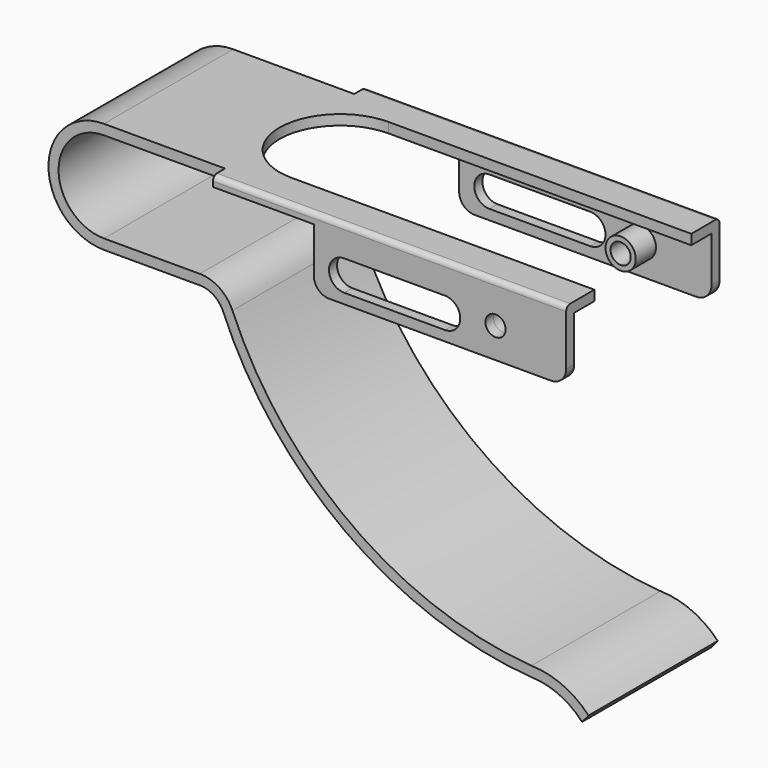
from build123d import *

# Parameters (mm, degrees)
F1_DEPTH  = 16
F2_W      = 70
F2_H      = 3
F3_DEPTH  = 2
F4_W      = 50
F4_H      = 14
F5_DEPTH  = 2
F6_R      = 1
F9_DEPTH  = 2
F11_DEPTH = 38.001
F13_D     = 4
F14_R     = 3
F14_R_2   = 2
F15_DEPTH = 5
F16_R     = 3


# Not quite as in the source:
# - a pattern or mirror of a feature is missing from the dataset's text; its kind, count and spacing are read off the source's solid


with BuildPart() as f1:
    # F0 (on Front) → F1 (new body)
    with BuildSketch(Plane.XZ):
        with BuildLine():
            Line((94, 11), (0, 11))
            ThreePointArc((0, 11), (-11, 0), (0, -11))
            Line((0, -11), (19, -11))
            ThreePointArc((19, -11), (21.7681124643, -11.8361612201), (23.6103896104, -14.064978646))
            ThreePointArc((23.6103896104, -14.064978646), (47.9223026847, -44.6255578719), (84.6125434697, -57.9988278946))
            ThreePointArc((84.6125434697, -57.9988278946), (90.1511361286, -59.2227601314), (94.7495356371, -62.543714922))
            Line((94.7495356371, -62.543714922), (96.0448662588, -61))
            ThreePointArc((96.0448662588, -61), (90.8779784788, -57.357163598), (84.7034264019, -56))
            ThreePointArc((84.7034264019, -56), (49.0672193413, -42.9854179344), (25.4545454545, -13.2909701044))
            ThreePointArc((25.4545454545, -13.2909701044), (22.87535745, -10.1706257081), (19, -9))
            Line((19, -9), (0, -9))
            ThreePointArc((0, -9), (-9, 0), (0, 9))
            Line((0, 9), (94, 9))
            Line((94, 9), (94, 11))
        make_face()
    extrude(amount=F1_DEPTH)

    # F2 (on face) → F3 (join)
    with BuildSketch(Plane.XY.offset(11)):
        with Locations((59, -17.5)):
            Rectangle(F2_W, F2_H)
    extrude(amount=-F3_DEPTH)

    # F4 (on face) → F5 (join)
    with BuildSketch(Plane.XZ.offset(19)):
        with Locations((69, 4)):
            Rectangle(F4_W, F4_H)
    extrude(amount=-F5_DEPTH)

    # F6
    f6_edges = [f1.edges().sort_by_distance(p)[0] for p in [
        (59, -19, 11),
    ]]
    fillet(f6_edges, radius=F6_R)

    # F7: F1 across plane


with BuildPart() as f1_1:
    add(f1.part)
    add(f1.part.mirror(Plane.XZ))

    # F8 (on face) → F9 (cut)
    with BuildSketch(Plane.XY.offset(11)):
        with BuildLine():
            Line((94, 12), (34, 12))
            ThreePointArc((34, 12), (22, 0), (34, -12))
            Line((34, -12), (94, -12))
            Line((94, -12), (94, 12))
        make_face()
    extrude(amount=-F9_DEPTH, mode=Mode.SUBTRACT)

    # F10 (on face) → F11 (cut, through all)
    with BuildSketch(Plane.XZ.offset(19)):
        with BuildLine():
            ThreePointArc((50, 5), (47, 2), (50, -1))
            Line((50, -1), (70, -1))
            ThreePointArc((70, -1), (73, 2), (70, 5))
            Line((70, 5), (50, 5))
        make_face()
    extrude(amount=-F11_DEPTH, mode=Mode.SUBTRACT)

    # F13 (through all)
    with Locations(Plane.XZ.offset(19)):
        with Locations((80, 3)):
            Hole(F13_D / 2)

    # F14 (on face) → F15 (join)
    with BuildSketch(Plane(origin=(0, -17, 0), x_dir=(-1, 0, 0), z_dir=(0, 1, 0))):
        with Locations((-80, 3)):
            Circle(F14_R)
        with Locations((-80, 3)):
            Circle(F14_R_2, mode=Mode.SUBTRACT)
    f15 = extrude(amount=F15_DEPTH)

    # F15_copies: F15 across plane
    add(f15.mirror(Plane.ZX))

    # F16
    f16_edges = [f1_1.edges().sort_by_distance(p)[0] for p in [
        (94, 18, -3),
        (44, 18, -3),
        (44, -18, -3),
        (94, -18, -3),
    ]]
    fillet(f16_edges, radius=F16_R)


solid = f1_1.part
